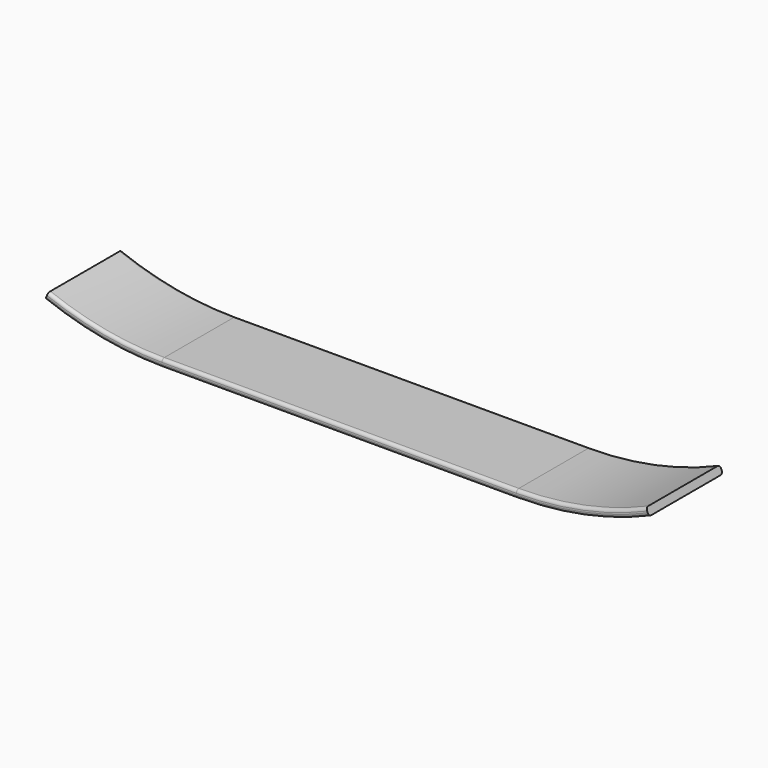
from build123d import *

# Parameters (mm, degrees)
F1_DEPTH = 76.2
F2_R     = 5.08
F3_R     = 5.08


# Not quite as in the source:
# - ends of sketch curves that miss each other by under 0.0002 mm in the source are joined


with BuildPart() as f1:
    # F0 (on Front) → F1 (new body, symmetric)
    with BuildSketch(Plane.XZ):
        with BuildLine():
            ThreePointArc((-192.4629807472, 35.8584225178), (-97.8874678184, 9.0410803069), (0, 0))
            Line((0, 0), (584.2, 0))
            ThreePointArc((584.2, 0), (695.6968250703, 11.3447270597), (802.6236891747, 44.9139177799))
            Line((802.6236891747, 44.9139177799), (797.6126335298, 56.5835017731))
            ThreePointArc((797.6126335298, 56.5835017731), (693.1388754415, 23.7844522554), (584.2, 12.6999948523))
            Line((584.2, 12.6999948523), (0, 12.7))
            ThreePointArc((0, 12.7), (-95.5613173512, 21.5262322224), (-187.8893835079, 47.7063000762))
            Line((-187.8893835079, 47.7063000762), (-192.4629807472, 35.8584225178))
        make_face()
    extrude(amount=F1_DEPTH, both=True)

    # F2
    f2_edges = [f1.edges().sort_by_distance(p)[0] for p in [
        (292.1, 76.2, 0),
        (292.1, 76.2, 12.699997),
    ]]
    fillet(f2_edges, radius=F2_R)

    # F3
    f3_edges = [f1.edges().sort_by_distance(p)[0] for p in [
        (292.1, -76.2, 0),
        (292.1, -76.2, 12.699997),
    ]]
    fillet(f3_edges, radius=F3_R)


solid = f1.part
